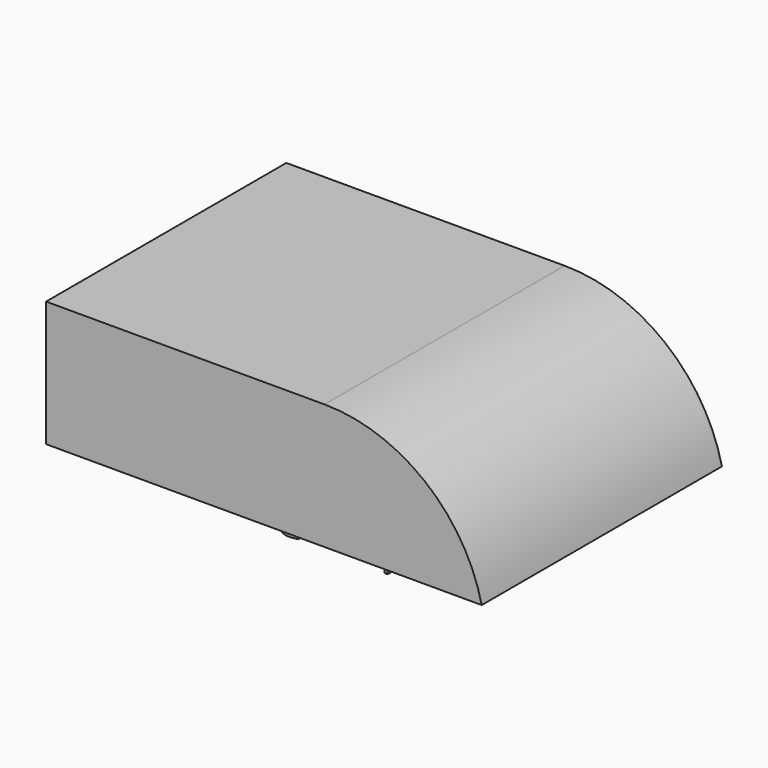
from build123d import *

# Parameters (mm, degrees)
F0_W          = 86.7475513369
F0_H          = 59.7936529666
F1_DEPTH      = 25
F2_T1_DEPTH   = 216.3545052716
F3_W          = 39.2890591174
F3_H          = 39.9312116206
F4_DEPTH      = 25
F5_DEPTH      = 28.5
F6_W          = 5.1124766469
F6_H          = 7.6591288671
F7_DEPTH      = 2
F8_R          = 7.5030248256
F9_DEPTH      = 1.2
F10_W         = 5.3160339594
F10_H         = 16.0010531545
F11_DEPTH     = 2
F12_TEXT_SIZE = 7.8950905138
F13_DEPTH     = 2.2


# Not quite as in the source:
# - a fillet or chamfer that OpenCascade refuses, or shapes differently, is made with other operations: its cross-section is extruded or revolved along the edge and cut away or added
# - Text() gives the source's letters only with a copy of the font that has no kerning and outlines rounded to 1/6400 em; it was checked with that copy


with BuildPart() as f1:
    # F0 (on Top) → F1 (new body)
    with BuildSketch(Plane.XY):
        with Locations((-63.559810631, 2.3034093902)):
            Rectangle(F0_W, F0_H)
    extrude(amount=F1_DEPTH)

    # F2: fillet of radius 32.1090403796 on 1 edges, made by hand

    # F2_s2 → F2_t1 (cut)
    with BuildSketch(Plane.XZ.offset(-110.4806620259)):
        with BuildLine():
            ThreePointArc((-20.1860349625, 0), (-31.4641592834, 17.983338331), (-51.4982054235, 25))
            Line((-51.4982054235, 25), (-20.1860349625, 25))
            Line((-20.1860349625, 25), (-20.1860349625, 0))
        make_face()
    extrude(amount=F2_T1_DEPTH, mode=Mode.SUBTRACT)

    # F3 (on face) → F4 (join)
    with BuildSketch(Plane(origin=(0, 0, 0), x_dir=(1, 0, 0), z_dir=(0, 0, -1))):
        with Locations((-50.0824218616, -3.0028745532)):
            Rectangle(F3_W, F3_H)
    extrude(amount=F4_DEPTH)

    # F5 (cut): a face of the model
    f5_faces = [f1.faces().sort_by_distance(p)[0] for p in [
        (-50.0824218616, 3.0028745532, -25),
    ]]
    extrude(f5_faces, amount=-F5_DEPTH, mode=Mode.SUBTRACT)

    # F6 (on face) → F7 (join)
    with BuildSketch(Plane(origin=(0, 0, 0), x_dir=(1, 0, 0), z_dir=(0, 0, -1))):
        with Locations((-78.7808932364, 17.8541061468)):
            Rectangle(F6_W, F6_H)
    extrude(amount=F7_DEPTH)

    # F8 (on face) → F9 (join)
    with BuildSketch(Plane(origin=(0, 0, 0), x_dir=(1, 0, 0), z_dir=(0, 0, -1))):
        with Locations((-77.8634026647, 0)):
            Circle(F8_R)
    extrude(amount=F9_DEPTH)

    # F10 (on face) → F11 (join)
    with BuildSketch(Plane(origin=(0, 0, 0), x_dir=(1, 0, 0), z_dir=(0, 0, -1))):
        with Locations((-79.0564492345, -21.217038855)):
            Rectangle(F10_W, F10_H)
    extrude(amount=F11_DEPTH)

    # F12 (on face) → F13 (join)
    with BuildSketch(Plane(origin=(0, 0, 0), x_dir=(1, 0, 0), z_dir=(0, 0, -1))):
        with Locations((-63.9549940825, 19.329611212)):
            Text('Gameboy', F12_TEXT_SIZE, font='Open Sans', text_align=(TextAlign.LEFT, TextAlign.BOTTOM))
    extrude(amount=F13_DEPTH)


solid = f1.part
